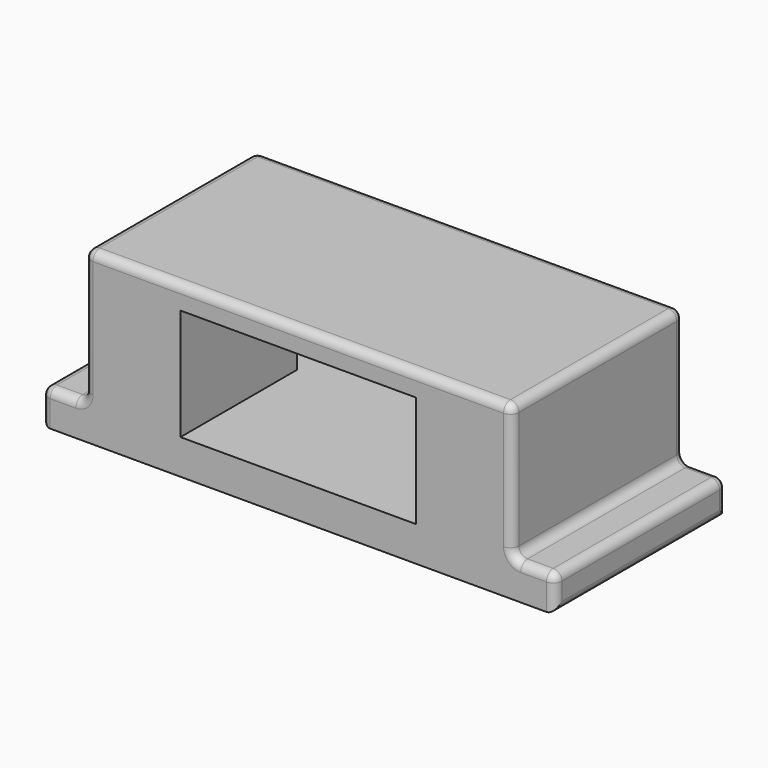
from build123d import *

# Parameters (mm, degrees)
F0_W     = 5
F0_H     = 4.0733553469
F0_W_2   = 6.2
F0_H_2   = 13
F1_DEPTH = 25
F2_DEPTH = 8
F3_R     = 1


with BuildPart() as f1:
    # F0 (on Front) → F1 (new body)
    with BuildSketch(Plane.XZ):
        with Locations((-13.7, -2.0366776735)):
            Rectangle(F0_W, F0_H)
        Polygon((38.7, 15.7062858343), (-11.2, 15.7062858343), (-11.2, 0), (-11.2, -4.0733553469), (38.7, -4.0733553469), (38.7, 0), align=None)
        Polygon((27.5, 0), (0, 0), (-6.2, 0), (-6.2, 13), (0, 13), (27.5, 13), (33.7, 13), (33.7, 0), align=None, mode=Mode.SUBTRACT)
        with Locations((41.2, -2.0366776735)):
            Rectangle(F0_W, F0_H)
        with Locations((-3.1, 6.5)):
            Rectangle(F0_W_2, F0_H_2)
        with Locations((30.6, 6.5)):
            Rectangle(F0_W_2, F0_H_2)
    extrude(amount=F1_DEPTH)

    # F0 (on Front) → F2 (cut)
    with BuildSketch(Plane.XZ):
        with Locations((30.6, 6.5)):
            Rectangle(F0_W_2, F0_H_2)
        with Locations((-3.1, 6.5)):
            Rectangle(F0_W_2, F0_H_2)
    extrude(amount=F2_DEPTH, mode=Mode.SUBTRACT)

    # F3
    f3_edges = [f1.edges().sort_by_distance(p)[0] for p in [
        (38.7, -12.5, 15.706286),
        (-11.2, -12.5, 15.706286),
        (13.75, 0, 15.706286),
        (13.75, -25, 15.706286),
        (38.7, -12.5, 0),
        (38.7, 0, 7.853143),
        (38.7, -25, 7.853143),
        (43.7, -12.5, 0),
        (41.2, 0, 0),
        (41.2, -25, 0),
        (43.7, -12.5, -4.073355),
        (43.7, 0, -2.036678),
        (43.7, -25, -2.036678),
        (-11.2, -12.5, 0),
        (-11.2, 0, 7.853143),
        (-11.2, -25, 7.853143),
        (-16.2, -12.5, 0),
        (-16.2, -12.5, -4.073355),
        (-16.2, 0, -2.036678),
        (-16.2, -25, -2.036678),
        (-13.7, 0, 0),
        (-13.7, -25, 0),
    ]]
    fillet(f3_edges, radius=F3_R)


solid = f1.part
